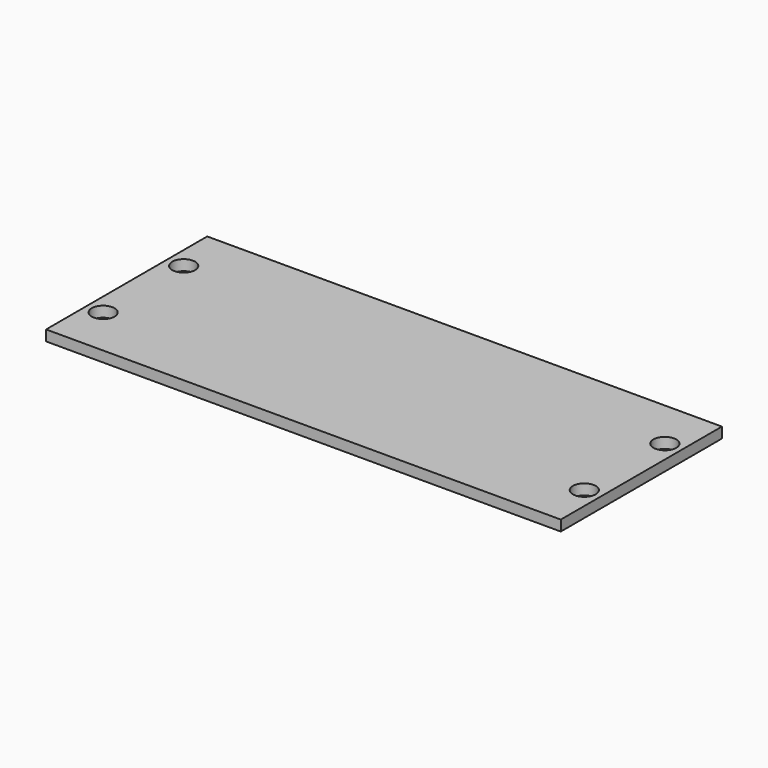
from build123d import *

# Parameters (mm, degrees)
F0_W     = 146.05
F0_H     = 57.15
F0_R     = 3.24
F1_DEPTH = 3


# Not quite as in the source:
# - ends of sketch curves that miss each other by under 0.0002 mm in the source are joined


with BuildPart() as f1:
    # F0 (on Top) → F1 (new body)
    with BuildSketch(Plane.XY):
        Rectangle(F0_W, F0_H)
        with Locations((-68.262, -14.287)):
            Circle(F0_R, mode=Mode.SUBTRACT)
        with Locations((68.262, -14.287)):
            Circle(F0_R, mode=Mode.SUBTRACT)
        with Locations((-68.262, 14.287)):
            Circle(F0_R, mode=Mode.SUBTRACT)
        with BuildLine():
            ThreePointArc((-68.262, 7.937), (-61.912, 14.287), (-68.262, 20.637))
            Line((-68.262, 20.637), (-72.225, 20.637))
            Line((-72.225, 20.637), (-72.225, 27.775))
            Line((-72.225, 27.775), (72.225, 27.775))
            Line((72.225, 27.775), (72.225, 20.636958))
            Line((72.225, 20.636958), (69.238962, 20.636958))
            ThreePointArc((69.238962, 20.636958), (62.9120417914, 14.2639619992), (69.2850380008, 7.9370417914))
            Line((69.2850380008, 7.9370417914), (72.225, 7.937042))
            Line((72.225, 7.937042), (72.225, -7.937576))
            Line((72.225, -7.937576), (68.176478, -7.937576))
            ThreePointArc((68.176478, -7.937576), (61.9125759326, -14.3725220009), (68.3475220009, -20.6364240674))
            Line((68.3475220009, -20.6364240674), (72.225, -20.636424))
            Line((72.225, -20.636424), (72.225, -27.775))
            Line((72.225, -27.775), (-72.225, -27.775))
            Line((-72.225, -27.775), (-72.225, -20.636871))
            Line((-72.225, -20.636871), (-69.221508, -20.636871))
            ThreePointArc((-69.221508, -20.636871), (-62.9121291038, -14.2465080007), (-69.3024919993, -7.9371291038))
            Line((-69.3024919993, -7.9371291038), (-72.225, -7.937129))
            Line((-72.225, -7.937129), (-72.225, 7.937))
            Line((-72.225, 7.937), (-68.262, 7.937))
        make_face(mode=Mode.SUBTRACT)
        with Locations((68.262, 14.287)):
            Circle(F0_R, mode=Mode.SUBTRACT)
        with BuildLine():
            Line((-72.225, 20.637), (-68.262, 20.637))
            ThreePointArc((-68.262, 20.637), (-61.912, 14.287), (-68.262, 7.937))
            Line((-68.262, 7.937), (-72.225, 7.937))
            Line((-72.225, 7.937), (-72.225, -7.937129))
            Line((-72.225, -7.937129), (-69.302492, -7.937129))
            ThreePointArc((-69.302492, -7.937129), (-62.9121291038, -14.2465080007), (-69.2215080007, -20.6368708962))
            Line((-69.2215080007, -20.6368708962), (-72.225, -20.636871))
            Line((-72.225, -20.636871), (-72.225, -27.775))
            Line((-72.225, -27.775), (72.225, -27.775))
            Line((72.225, -27.775), (72.225, -20.636424))
            Line((72.225, -20.636424), (68.347522, -20.636424))
            ThreePointArc((68.347522, -20.636424), (61.9125759326, -14.3725220009), (68.1764779991, -7.9375759326))
            Line((68.1764779991, -7.9375759326), (72.225, -7.937576))
            Line((72.225, -7.937576), (72.225, 7.937042))
            Line((72.225, 7.937042), (69.285038, 7.937042))
            ThreePointArc((69.285038, 7.937042), (62.9120417914, 14.2639619992), (69.2389619992, 20.6369582086))
            Line((69.2389619992, 20.6369582086), (72.225, 20.636958))
            Line((72.225, 20.636958), (72.225, 27.775))
            Line((72.225, 27.775), (-72.225, 27.775))
            Line((-72.225, 27.775), (-72.225, 20.637))
        make_face()
    extrude(amount=F1_DEPTH)


solid = f1.part
